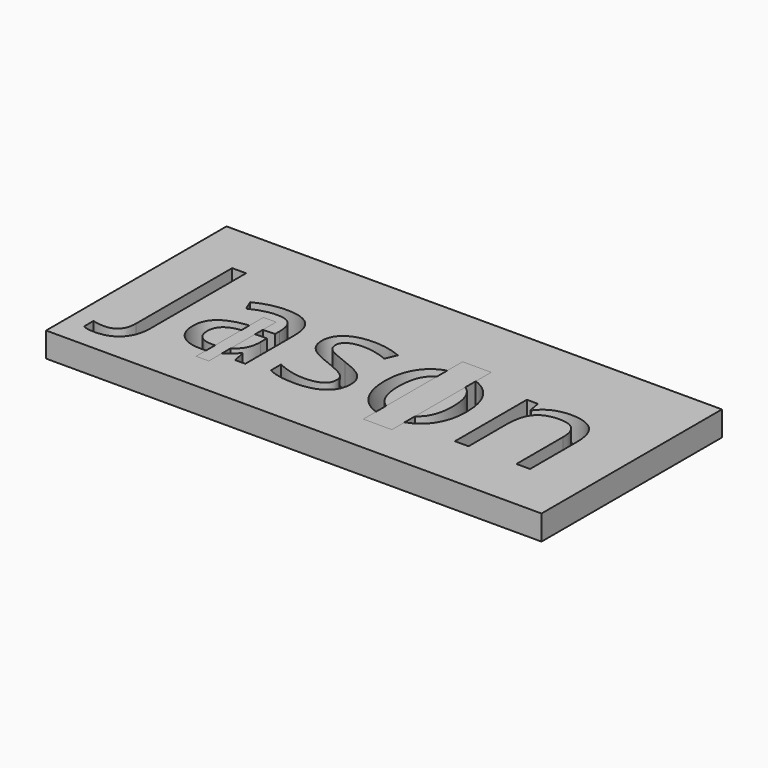
from build123d import *

# Parameters (mm, degrees)
F0_W         = 101.6
F0_H         = 46.2507452278
F1_DEPTH     = 5.08
F2_TEXT_SIZE = 34.451105056
F3_DEPTH     = 25.4
F5_DEPTH     = 5.08


# Not quite as in the source:
# - Text() gives the source's letters only with a copy of the font that has no kerning and outlines rounded to 1/6400 em; it was checked with that copy


with BuildPart() as f1:
    # F0 (on Top) → F1 (new body)
    with BuildSketch(Plane.XY):
        Rectangle(F0_W, F0_H)
    extrude(amount=F1_DEPTH)

    # F2 (on face) → F3 (cut)
    with BuildSketch(Plane.XY.offset(5.08)):
        with Locations((-44.2483602991, -12.2156894252)):
            Text('Jason', F2_TEXT_SIZE, font='Open Sans', text_align=(TextAlign.LEFT, TextAlign.BOTTOM))
    extrude(amount=-F3_DEPTH, mode=Mode.SUBTRACT)


with BuildPart() as f5:
    # F4 (on face) → F5 (new body)
    with BuildSketch(Plane.XY.offset(5.08)):
        with BuildLine():
            Line((-26.4577753842, -1.3973150955), (-26.4577753842, -12.500818706))
            add(Edge.make_bspline(
                [(-26.4577753842, -12.500818706), (-25.1531378895, -12.3723832609), (-24.0204181598, -11.8627706517), (-23.8520484534, -11.7702287621)],
                knots=[2.0371406811, 2.0371406811, 2.0371406811, 2.2837393645, 2.3267574348, 2.3267574348, 2.3267574348], degree=2))
            Line((-23.8520484534, -11.7702287621), (-23.8520484534, -1.24433515))
            Line((-23.8520484534, -1.24433515), (-24.5358686248, -1.2666975996))
            add(Edge.make_bspline(
                [(-24.5358686248, -1.2666975996), (-25.5549700699, -1.2974119289), (-26.4577753842, -1.3973150955)],
                knots=[0, 0, 0, 0.1141163437, 0.1141163437, 0.1141163437], degree=2))
        make_face()
        with BuildLine():
            Line((-26.4577753842, 2.1605324), (-26.4577753842, -1.3973150955))
            add(Edge.make_bspline(
                [(-24.5358686248, -1.2666975996), (-25.5549700699, -1.2974119289), (-26.4577753842, -1.3973150955)],
                knots=[0, 0, 0, 0.1141163437, 0.1141163437, 0.1141163437], degree=2))
            Line((-24.5358686248, -1.2666975996), (-23.8520484534, -1.24433515))
            Line((-23.8520484534, -1.24433515), (-23.8520484534, 2.1605324))
            Line((-23.8520484534, 2.1605324), (-26.4577753842, 2.1605324))
        make_face()
        with BuildLine():
            Line((-26.4577753842, -12.500818706), (-26.4577753842, -15.1085611433))
            Line((-26.4577753842, -15.1085611433), (-23.8520484534, -15.1085611433))
            Line((-23.8520484534, -15.1085611433), (-23.8520484534, -11.7702287621))
            add(Edge.make_bspline(
                [(-26.4577753842, -12.500818706), (-25.1531378895, -12.3723832609), (-24.0204181598, -11.8627706517), (-23.8520484534, -11.7702287621)],
                knots=[2.0371406811, 2.0371406811, 2.0371406811, 2.2837393645, 2.3267574348, 2.3267574348, 2.3267574348], degree=2))
        make_face()
    extrude(amount=-F5_DEPTH)


with BuildPart() as f5b:
    # F4 (on face) → F5, piece 2 (new body)
    with BuildSketch(Plane.XY.offset(5.08)):
        with BuildLine():
            add(Edge.make_bspline(
                [(13.9274941757, 6.1163025004), (12.5962540678, 6.5601628303), (9.3828117481, 6.5601628303), (8.0561727526, 6.1539661476)],
                knots=[1.5848829196, 1.5848829196, 1.5848829196, 2, 2.4163075416, 2.4163075416, 2.4163075416], degree=2))
            Line((13.9274941757, 6.1163025004), (13.9274941757, 10.0760553032))
            Line((13.9274941757, 10.0760553032), (8.0561727526, 10.0760553032))
            Line((8.0561727526, 10.0760553032), (8.0561727526, 6.1539661476))
        make_face()
        with BuildLine():
            add(Edge.make_bspline(
                [(8.0561727526, -12.1206320917), (9.360264157, -12.5548174906), (12.5531412765, -12.5548174906), (13.9274941757, -12.1092932549)],
                knots=[5.672429471, 5.672429471, 5.672429471, 6.0817084494, 6.5360470791, 6.5360470791, 6.5360470791], degree=2))
            Line((13.9274941757, -12.1092932549), (13.9274941757, 6.1163025004))
            add(Edge.make_bspline(
                [(13.9274941757, 6.1163025004), (12.5962540678, 6.5601628303), (9.3828117481, 6.5601628303), (8.0561727526, 6.1539661476)],
                knots=[1.5848829196, 1.5848829196, 1.5848829196, 2, 2.4163075416, 2.4163075416, 2.4163075416], degree=2))
            Line((8.0561727526, 6.1539661476), (8.0561727526, -12.1206320917))
        make_face()
        with BuildLine():
            Line((8.0561727526, -15.3837827966), (13.9274941757, -15.3837827966))
            Line((13.9274941757, -15.3837827966), (13.9274941757, -12.1092932549))
            add(Edge.make_bspline(
                [(8.0561727526, -12.1206320917), (9.360264157, -12.5548174906), (12.5531412765, -12.5548174906), (13.9274941757, -12.1092932549)],
                knots=[5.672429471, 5.672429471, 5.672429471, 6.0817084494, 6.5360470791, 6.5360470791, 6.5360470791], degree=2))
            Line((8.0561727526, -12.1206320917), (8.0561727526, -15.3837827966))
        make_face()
    extrude(amount=-F5_DEPTH)


solid = Compound([f1.part, f5.part, f5b.part])
